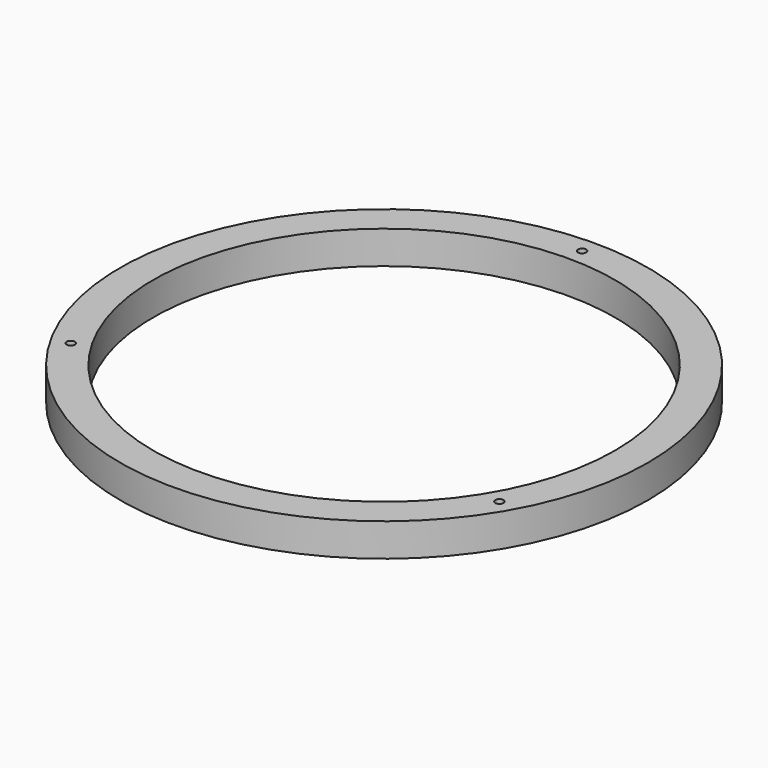
from build123d import *

# Parameters (mm, degrees)
F0_R     = 2438.4
F0_R_2   = 38.1
F0_R_3   = 2133.6
F1_DEPTH = 304.8


# Not quite as in the source:
# - a feature names something its author has since deleted; it is built from what else it names


with BuildPart() as f1:
    # F0 (on Top) → F1 (new body)
    with BuildSketch(Plane.XY):
        Circle(F0_R)
        with Locations((-1979.7340730512, -1143)):
            Circle(F0_R_2, mode=Mode.SUBTRACT)
        with Locations((1979.7340730512, -1143)):
            Circle(F0_R_2, mode=Mode.SUBTRACT)
        Circle(F0_R_3, mode=Mode.SUBTRACT)
        with Locations((0, 2286)):
            Circle(F0_R_2, mode=Mode.SUBTRACT)
    extrude(amount=F1_DEPTH)


solid = f1.part
